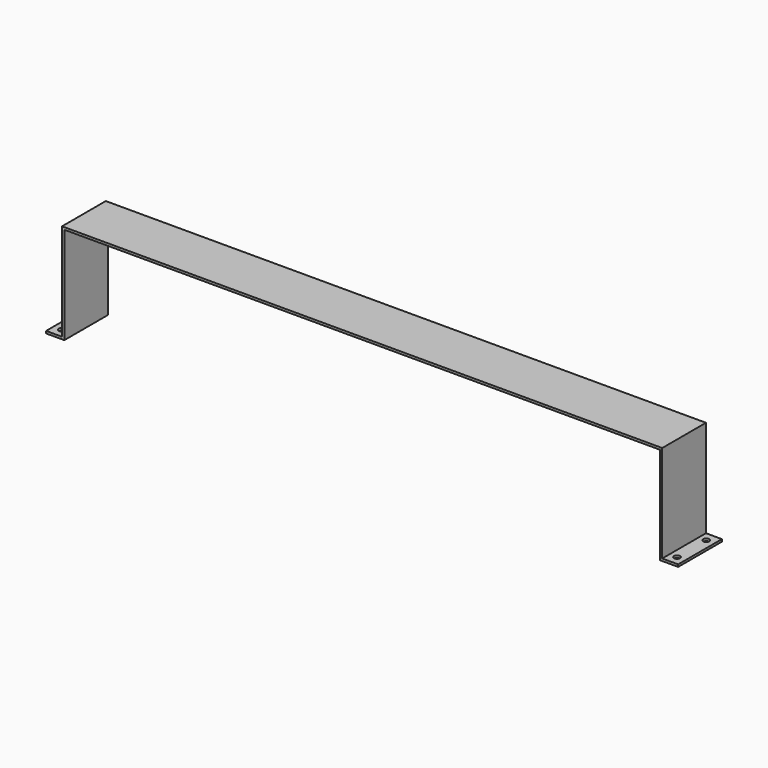
from build123d import *

# Parameters (mm, degrees)
F1_DEPTH = 57.15
F3_D     = 12.7


# Not quite as in the source:
# - a length typed as a fraction of an inch, garbled in the dataset ("3 / 203.2 mm" for 3/8 in), is restored


with BuildPart() as f1:
    # F0 (on Front) → F1 (new body, symmetric)
    with BuildSketch(Plane.XZ):
        Polygon((-627.0625, 4.7625), (-660.4, 4.7625), (-660.4, 0), (-622.3, 0), (-622.3, 203.2), (622.3, 203.2), (622.3, 0), (660.4, 0), (660.4, 4.7625), (627.0625, 4.7625), (627.0625, 207.9625), (-627.0625, 207.9625), align=None)
    extrude(amount=F1_DEPTH, both=True)

    # F3 (through all)
    with Locations(Plane.XY.offset(4.7625)):
        with Locations((-642.9375, 38.1), (-642.9375, -38.1), (642.9375, 38.1), (642.9375, -38.1)):
            Hole(F3_D / 2)


solid = f1.part
